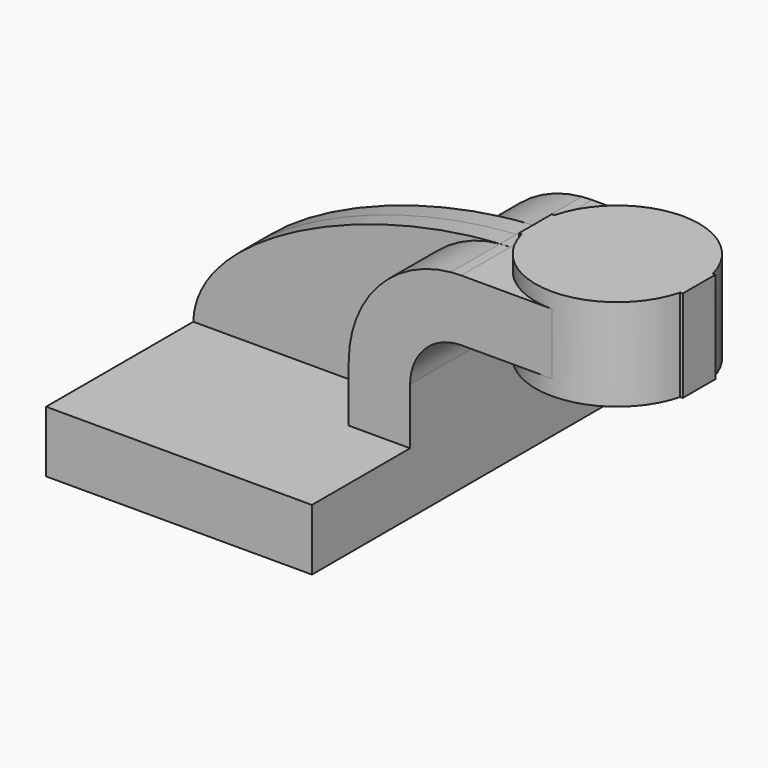
from build123d import *

# Parameters (mm, degrees)
F1_DEPTH = 63.5
F0_W     = 25.4
F0_H     = 19.05
F2_DEPTH = 25.4
F0_H_2   = 4.7498
F0_H_3   = 4.7752
F3_DEPTH = 6.35


with BuildPart() as f1:
    # F0 (on Front) → F1 (new body, symmetric)
    with BuildSketch(Plane.XZ):
        Polygon((22.225, 9.525), (-41.275, 9.525), (-41.275, -9.525), (41.275, -9.525), (41.275, 9.525), align=None)
    extrude(amount=F1_DEPTH, both=True)

    # F0 (on Front) → F2 (join, symmetric)
    with BuildSketch(Plane.XZ):
        with BuildLine():
            Line((22.225, 27.0002), (22.225, 9.525))
            Line((22.225, 9.525), (41.275, 9.525))
            Line((41.275, 9.525), (41.275, 27.0002))
            ThreePointArc((41.275, 27.0002), (45.9246798487, 38.2255201513), (57.15, 42.8752))
            Line((57.15, 42.8752), (59.9058770299, 42.8752))
            Line((59.9058770299, 42.8752), (59.9058770299, 61.9252))
            Line((59.9058770299, 61.9252), (57.15, 61.9252))
            add(Edge.make_bspline(
                [(53.9486358341, 61.7781656173), (55.0198111494, 61.8401017222), (56.0872015852, 61.8892118375), (57.15, 61.9252)],
                knots=[108.8616343251, 108.8616343251, 108.8616343251, 108.8616343251, 111.5045361635, 111.5045361635, 111.5045361635, 111.5045361635], degree=3))
            ThreePointArc((53.9486358341, 61.7781656173), (31.3472552962, 50.5368520719), (22.225, 27.0002))
        make_face()
        with Locations((72.6058770299, 52.4002)):
            Rectangle(F0_W, F0_H)
    extrude(amount=F2_DEPTH, both=True)

    # F0 (on Front) → F3 (join, symmetric)
    with BuildSketch(Plane.XZ):
        with BuildLine():
            add(Edge.make_bspline(
                [(-41.275, 9.525), (-40.7167454474, 34.9148619979), (9.8267188659, 59.2270055586), (53.9486358341, 61.7781656173)],
                knots=[0, 0, 0, 0, 108.8616343251, 108.8616343251, 108.8616343251, 108.8616343251], degree=3))
            Line((-41.275, 9.525), (22.225, 9.525))
            Line((22.225, 9.525), (22.225, 27.0002))
            ThreePointArc((22.225, 27.0002), (31.3472552962, 50.5368520719), (53.9486358341, 61.7781656173))
        make_face()
        Polygon((22.225, 9.525), (-41.275, 9.525), (-41.275, -9.525), (41.275, -9.525), (41.275, 9.525), align=None)
        with BuildLine():
            Line((22.225, 27.0002), (22.225, 9.525))
            Line((22.225, 9.525), (41.275, 9.525))
            Line((41.275, 9.525), (41.275, 27.0002))
            ThreePointArc((41.275, 27.0002), (45.9246798487, 38.2255201513), (57.15, 42.8752))
            Line((57.15, 42.8752), (59.9058770299, 42.8752))
            Line((59.9058770299, 42.8752), (59.9058770299, 61.9252))
            Line((59.9058770299, 61.9252), (57.15, 61.9252))
            add(Edge.make_bspline(
                [(53.9486358341, 61.7781656173), (55.0198111494, 61.8401017222), (56.0872015852, 61.8892118375), (57.15, 61.9252)],
                knots=[108.8616343251, 108.8616343251, 108.8616343251, 108.8616343251, 111.5045361635, 111.5045361635, 111.5045361635, 111.5045361635], degree=3))
            ThreePointArc((53.9486358341, 61.7781656173), (31.3472552962, 50.5368520719), (22.225, 27.0002))
        make_face()
        with BuildLine():
            ThreePointArc((57.15, 61.9252), (55.5476305332, 61.8884220397), (53.9486358341, 61.7781656173))
            add(Edge.make_bspline(
                [(53.9486358341, 61.7781656173), (55.0198111494, 61.8401017222), (56.0872015852, 61.8892118375), (57.15, 61.9252)],
                knots=[108.8616343251, 108.8616343251, 108.8616343251, 108.8616343251, 111.5045361635, 111.5045361635, 111.5045361635, 111.5045361635], degree=3))
        make_face()
        with Locations((72.6058770299, 52.4002)):
            Rectangle(F0_W, F0_H)
        with Locations((72.6058770299, 64.3001)):
            Rectangle(F0_W, F0_H_2)
        with Locations((72.6058770299, 40.4876)):
            Rectangle(F0_W, F0_H_3)
        Polygon((85.3058770299, 66.675), (85.3058770299, 61.9252), (85.3058770299, 42.8752), (85.3058770299, 38.1), (110.7058770299, 38.1), (110.7058770299, 66.675), align=None)
    extrude(amount=F3_DEPTH, both=True)

    # F0 (on Front) → F4 (revolve)
    with BuildSketch(Plane.XZ):
        Polygon((85.3058770299, 66.675), (85.3058770299, 61.9252), (85.3058770299, 42.8752), (85.3058770299, 38.1), (110.7058770299, 38.1), (110.7058770299, 66.675), align=None)
    revolve(axis=Axis((85.3058770299, 0, 52.3875), (0, 0, 1)))


solid = f1.part
